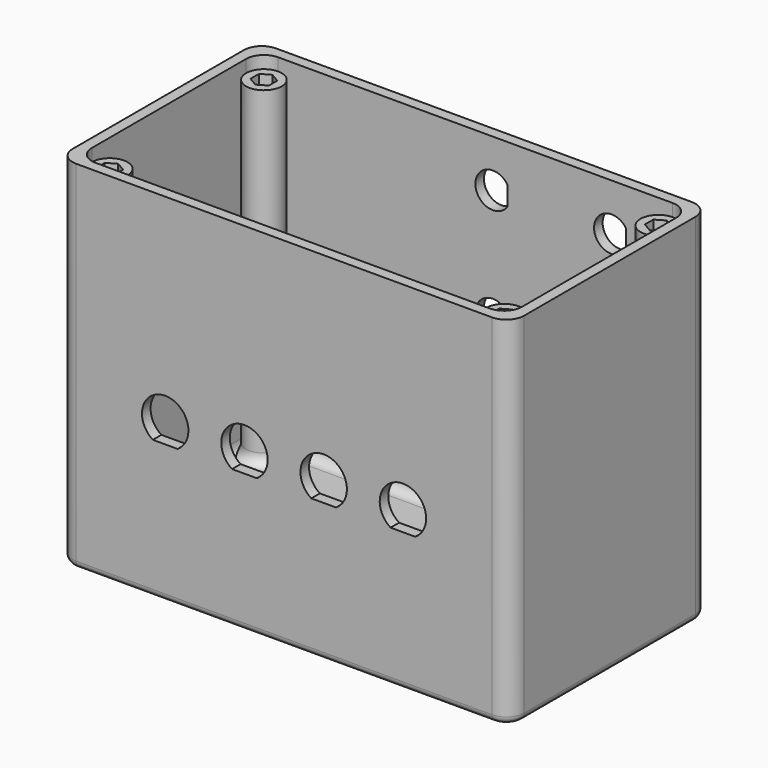
from build123d import *

# Parameters (mm, degrees)
F1_DEPTH      = 100
F3_DEPTH      = 96
F4_R          = 2
F5_R          = 5
F6_DEPTH      = 92.5
F8_DEPTH      = 12.5
F9_TEXT_SIZE  = 19.5676766441
F10_DEPTH     = 1.5
F12_DEPTH     = 25
F14_DEPTH     = 25
F15_T1_DEPTH  = 125.5
F15_T3_DEPTH  = 69
F15_T6_ANGLE  = 359.64
F15_T8_ANGLE  = 359.64
F15_T10_ANGLE = 359.64
F15_T12_ANGLE = 359.64


# Not quite as in the source:
# - a fillet or chamfer that OpenCascade refuses, or shapes differently, is made with other operations: its cross-section is extruded or revolved along the edge and cut away or added
# - Text() gives the source's letters only with a copy of the font that has no kerning and outlines rounded to 1/6400 em; it was checked with that copy


with BuildPart() as f1:
    # F0 (on Top) → F1 (new body)
    with BuildSketch(Plane.XY):
        with BuildLine():
            Line((-58.25, -35), (58.25, -35))
            ThreePointArc((58.25, -35), (61.7855339059, -33.5355339059), (63.25, -30))
            Line((63.25, -30), (63.25, 30))
            ThreePointArc((63.25, 30), (61.7855339059, 33.5355339059), (58.25, 35))
            Line((58.25, 35), (-58.25, 35))
            ThreePointArc((-58.25, 35), (-61.7855339059, 33.5355339059), (-63.25, 30))
            Line((-63.25, 30), (-63.25, -30))
            ThreePointArc((-63.25, -30), (-61.7855339059, -33.5355339059), (-58.25, -35))
        make_face()
    extrude(amount=F1_DEPTH)

    # F2 (on face) → F3 (cut)
    with BuildSketch(Plane.XY.offset(100)):
        with BuildLine():
            ThreePointArc((60.25, 27), (58.7855339059, 30.5355339059), (55.25, 32))
            Line((55.25, 32), (-55.25, 32))
            ThreePointArc((-55.25, 32), (-58.7855339059, 30.5355339059), (-60.25, 27))
            Line((-60.25, 27), (-60.25, -27))
            ThreePointArc((-60.25, -27), (-58.7855339059, -30.5355339059), (-55.25, -32))
            Line((-55.25, -32), (55.25, -32))
            ThreePointArc((55.25, -32), (58.7855339059, -30.5355339059), (60.25, -27))
            Line((60.25, -27), (60.25, 27))
        make_face()
    extrude(amount=-F3_DEPTH, mode=Mode.SUBTRACT)

    # F4
    f4_edges = [f1.edges().sort_by_distance(p)[0] for p in [
        (63.25, 0, 0),
        (61.785534, -33.535534, 0),
        (0, -35, 0),
        (61.785534, 33.535534, 0),
        (0, 35, 0),
        (-61.785534, 33.535534, 0),
        (-63.25, 0, 0),
        (-61.785534, -33.535534, 0),
    ]]
    fillet(f4_edges, radius=F4_R)

    # F5 (on face) → F6 (join)
    with BuildSketch(Plane.XY.offset(4)):
        with Locations((-55.25, 27)):
            Circle(F5_R)
        with Locations((55.25, 27)):
            Circle(F5_R)
        with Locations((-55.25, -27)):
            Circle(F5_R)
        with Locations((55.25, -27)):
            Circle(F5_R)
    extrude(amount=F6_DEPTH)

    # F7 (on face) → F8 (cut)
    with BuildSketch(Plane.XY.offset(96.5)):
        Polygon((-55.25, 24.020872611), (-52.67, 25.5104363055), (-52.67, 28.4895636945), (-55.25, 29.979127389), (-57.83, 28.4895636945), (-57.83, 25.5104363055), align=None)
        Polygon((57.83, 25.5104363055), (57.83, 28.4895636945), (55.25, 29.979127389), (52.67, 28.4895636945), (52.67, 25.5104363055), (55.25, 24.020872611), align=None)
        Polygon((-55.25, -24.020872611), (-57.83, -25.5104363055), (-57.83, -28.4895636945), (-55.25, -29.979127389), (-52.67, -28.4895636945), (-52.67, -25.5104363055), align=None)
        Polygon((55.25, -29.979127389), (57.83, -28.4895636945), (57.83, -25.5104363055), (55.25, -24.020872611), (52.67, -25.5104363055), (52.67, -28.4895636945), align=None)
    extrude(amount=-F8_DEPTH, mode=Mode.SUBTRACT)

    # F9 (on face) → F10 (cut)
    with BuildSketch(Plane(origin=(0, 0, 0), x_dir=(1, 0, 0), z_dir=(0, 0, -1))):
        with Locations((-50.2364951971, -5.8856116755)):
            Text('Trescal A/S', F9_TEXT_SIZE, font='Open Sans', text_align=(TextAlign.LEFT, TextAlign.BOTTOM))
    extrude(amount=-F10_DEPTH, mode=Mode.SUBTRACT)

    # F11 (on face) → F12 (cut)
    with BuildSketch(Plane.XZ.offset(35)):
        with BuildLine():
            Line((-36.7641016151, 38.9), (-29.8358983849, 38.9))
            ThreePointArc((-29.8358983849, 38.9), (-33.3, 50.9), (-36.7641016151, 38.9))
        make_face()
        with BuildLine():
            Line((-14.5641016151, 38.9), (-7.6358983849, 38.9))
            ThreePointArc((-7.6358983849, 38.9), (-11.1, 50.9), (-14.5641016151, 38.9))
        make_face()
        with BuildLine():
            ThreePointArc((36.7641016151, 38.9), (33.3, 50.9), (29.8358983849, 38.9))
            Line((29.8358983849, 38.9), (36.7641016151, 38.9))
        make_face()
        with BuildLine():
            ThreePointArc((14.5641016151, 38.9), (11.1, 50.9), (7.6358983849, 38.9))
            Line((7.6358983849, 38.9), (14.5641016151, 38.9))
        make_face()
    extrude(amount=-F12_DEPTH, mode=Mode.SUBTRACT)

    # F13 (on face) → F14 (cut)
    with BuildSketch(Plane(origin=(0, 35, 0), x_dir=(-1, 0, 0), z_dir=(0, 1, 0))):
        with BuildLine():
            Line((-42.25, 89.433281573), (-42.25, 84.066718427))
            ThreePointArc((-42.25, 84.066718427), (-33.25, 86.75), (-42.25, 89.433281573))
        make_face()
        with BuildLine():
            Line((-42.25, 57.783281573), (-42.25, 52.416718427))
            ThreePointArc((-42.25, 52.416718427), (-33.25, 55.1), (-42.25, 57.783281573))
        make_face()
        with BuildLine():
            Line((-9, 57.783281573), (-9, 52.416718427))
            ThreePointArc((-9, 52.416718427), (0, 55.1), (-9, 57.783281573))
        make_face()
        with BuildLine():
            Line((-9, 89.433281573), (-9, 84.066718427))
            ThreePointArc((-9, 84.066718427), (0, 86.75), (-9, 89.433281573))
        make_face()
    extrude(amount=-F14_DEPTH, mode=Mode.SUBTRACT)

    # F15: fillet of radius 3 on 8 edges, made by hand

    # F15_s2 → F15_t1 (join)
    with BuildSketch(Plane.YZ.offset(-62.75)):
        with BuildLine():
            ThreePointArc((32, 7), (31.1213203436, 4.8786796564), (29, 4))
            Line((29, 4), (32, 4))
            Line((32, 4), (32, 7))
        make_face()
        with BuildLine():
            ThreePointArc((-32, 7), (-31.1213203436, 4.8786796564), (-29, 4))
            Line((-29, 4), (-32, 4))
            Line((-32, 4), (-32, 7))
        make_face()
    extrude(amount=F15_T1_DEPTH)

    # F15_s4 → F15_t3 (join)
    with BuildSketch(Plane.XZ.offset(-34.5)):
        with BuildLine():
            ThreePointArc((-60.25, 7), (-59.3713203436, 4.8786796564), (-57.25, 4))
            Line((-57.25, 4), (-60.25, 4))
            Line((-60.25, 4), (-60.25, 7))
        make_face()
        with BuildLine():
            ThreePointArc((60.25, 7), (59.3713203436, 4.8786796564), (57.25, 4))
            Line((57.25, 4), (60.25, 4))
            Line((60.25, 4), (60.25, 7))
        make_face()
    extrude(amount=F15_T3_DEPTH)

    # F15_s5 → F15_t6 (revolve)
    with BuildSketch(Plane(origin=(-13.9516946264, -14.0396322626, 0), x_dir=(0, 0, 1), z_dir=(0.7048818539, 0.7093247296, 0))):
        with BuildLine():
            ThreePointArc((4, -66.2220013653), (4.8786796564, -64.1006810218), (7, -63.2220013653))
            Line((7, -63.2220013653), (4, -63.2220013653))
            Line((4, -63.2220013653), (4, -66.2220013653))
        make_face()
    revolve(axis=Axis((-55.25, 27, 4), (0, 0, 1)), revolution_arc=F15_T6_ANGLE)

    # F15_s7 → F15_t8 (revolve)
    with BuildSketch(Plane(origin=(13.9516946264, 14.0396322626, 0), x_dir=(0, 0, 1), z_dir=(-0.7048818539, -0.7093247296, 0))):
        with BuildLine():
            ThreePointArc((4, -66.2220013653), (4.8786796564, -64.1006810218), (7, -63.2220013653))
            Line((7, -63.2220013653), (4, -63.2220013653))
            Line((4, -63.2220013653), (4, -66.2220013653))
        make_face()
    revolve(axis=Axis((55.25, -27, 4), (0, 0, 1)), revolution_arc=F15_T8_ANGLE)

    # F15_s9 → F15_t10 (revolve)
    with BuildSketch(Plane(origin=(-13.9516946264, 14.0396322626, 0), x_dir=(0, 0, 1), z_dir=(0.7048818539, -0.7093247296, 0))):
        with BuildLine():
            ThreePointArc((4, 66.2220013653), (4.8786796564, 64.1006810218), (7, 63.2220013653))
            Line((7, 63.2220013653), (4, 63.2220013653))
            Line((4, 63.2220013653), (4, 66.2220013653))
        make_face()
    revolve(axis=Axis((-55.25, -27, 4), (0, 0, -1)), revolution_arc=F15_T10_ANGLE)

    # F15_s11 → F15_t12 (revolve)
    with BuildSketch(Plane(origin=(14.2988383305, -14.2092771497, 0), x_dir=(0, 0, 1), z_dir=(0.7093247296, -0.7048818539, 0))):
        with BuildLine():
            ThreePointArc((7, -63.0964901288), (4.8786796564, -63.9751697852), (4, -66.0964901288))
            Line((4, -66.0964901288), (4, -63.0964901288))
            Line((4, -63.0964901288), (7, -63.0964901288))
        make_face()
    revolve(axis=Axis((55.25, 27, 4), (0, 0, 1)), revolution_arc=F15_T12_ANGLE)


solid = f1.part
